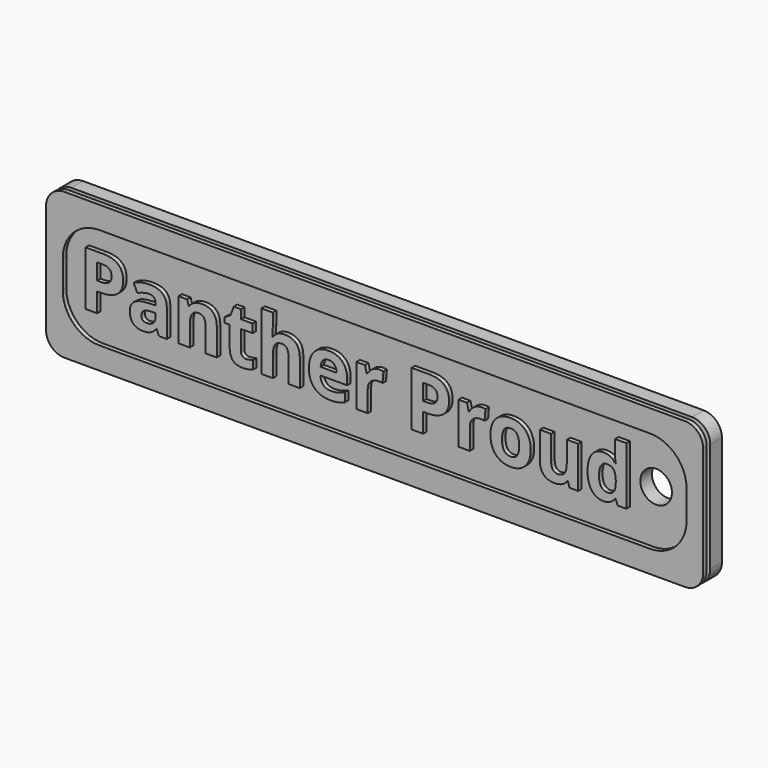
from build123d import *

# Parameters (mm, degrees)
F0_W         = 114.3
F0_H         = 25.4
F0_R         = 2.7522704915
F1_DEPTH     = 2.54
F2_TEXT_SIZE = 13.2291666667
F3_DEPTH     = 0.762
F4_R         = 3.175
F5_R         = 3.175
F6_R         = 3.175
F7_R         = 3.175
F9_DEPTH     = 0.762


# Not quite as in the source:
# - Text() gives the source's letters only with a copy of the font that has no kerning and outlines rounded to 1/6400 em; it was checked with that copy


with BuildPart() as f1:
    # F0 (on Front) → F1 (new body)
    with BuildSketch(Plane.XZ):
        Rectangle(F0_W, F0_H)
        with Locations((47.738853842, 0)):
            Circle(F0_R, mode=Mode.SUBTRACT)
    extrude(amount=F1_DEPTH)

    # F2 (on face) → F3 (join)
    with BuildSketch(Plane.XZ.offset(2.54)):
        with Locations((-52.0640315589, -4.5523742514)):
            Text('Panther Proud', F2_TEXT_SIZE, font='Open Sans', font_style=FontStyle.BOLD, text_align=(TextAlign.LEFT, TextAlign.BOTTOM))
    extrude(amount=F3_DEPTH)

    # F4
    f4_edges = [f1.edges().sort_by_distance(p)[0] for p in [
        (-57.15, -1.27, -12.7),
    ]]
    fillet(f4_edges, radius=F4_R)

    # F5
    f5_edges = [f1.edges().sort_by_distance(p)[0] for p in [
        (-57.15, -1.27, 12.7),
    ]]
    fillet(f5_edges, radius=F5_R)

    # F6
    f6_edges = [f1.edges().sort_by_distance(p)[0] for p in [
        (57.15, -1.27, 12.7),
    ]]
    fillet(f6_edges, radius=F6_R)

    # F7
    f7_edges = [f1.edges().sort_by_distance(p)[0] for p in [
        (57.15, -1.27, -12.7),
    ]]
    fillet(f7_edges, radius=F7_R)


with BuildPart() as f9:
    # F8 (on face) → F9 (new body)
    with BuildSketch(Plane.XZ.offset(3.302)):
        with BuildLine():
            ThreePointArc((57.15, 9.525), (56.2200640303, 11.7700640303), (53.975, 12.7))
            Line((53.975, 12.7), (-53.975, 12.7))
            ThreePointArc((-53.975, 12.7), (-56.2200640303, 11.7700640303), (-57.15, 9.525))
            Line((-57.15, 9.525), (-57.15, -9.525))
            ThreePointArc((-57.15, -9.525), (-56.2200640303, -11.7700640303), (-53.975, -12.7))
            Line((-53.975, -12.7), (53.975, -12.7))
            ThreePointArc((53.975, -12.7), (56.2200640303, -11.7700640303), (57.15, -9.525))
            Line((57.15, -9.525), (57.15, 9.525))
        make_face()
        with BuildLine():
            ThreePointArc((54.2502366006, -2.4793170556), (52.3903646612, -6.9694451162), (47.9002366006, -8.8293170556))
            Line((47.9002366006, -8.8293170556), (-47.9002366006, -8.8293170556))
            ThreePointArc((-47.9002366006, -8.8293170556), (-52.3903646612, -6.9694451162), (-54.2502366006, -2.4793170556))
            Line((-54.2502366006, -2.4793170556), (-54.2502366006, 2.4793170556))
            ThreePointArc((-54.2502366006, 2.4793170556), (-52.3903646612, 6.9694451162), (-47.9002366006, 8.8293170556))
            Line((-47.9002366006, 8.8293170556), (47.9002366006, 8.8293170556))
            ThreePointArc((47.9002366006, 8.8293170556), (52.3903646612, 6.9694451162), (54.2502366006, 2.4793170556))
            Line((54.2502366006, 2.4793170556), (54.2502366006, -2.4793170556))
        make_face(mode=Mode.SUBTRACT)
    extrude(amount=F9_DEPTH)


solid = Compound([f1.part, f9.part])
